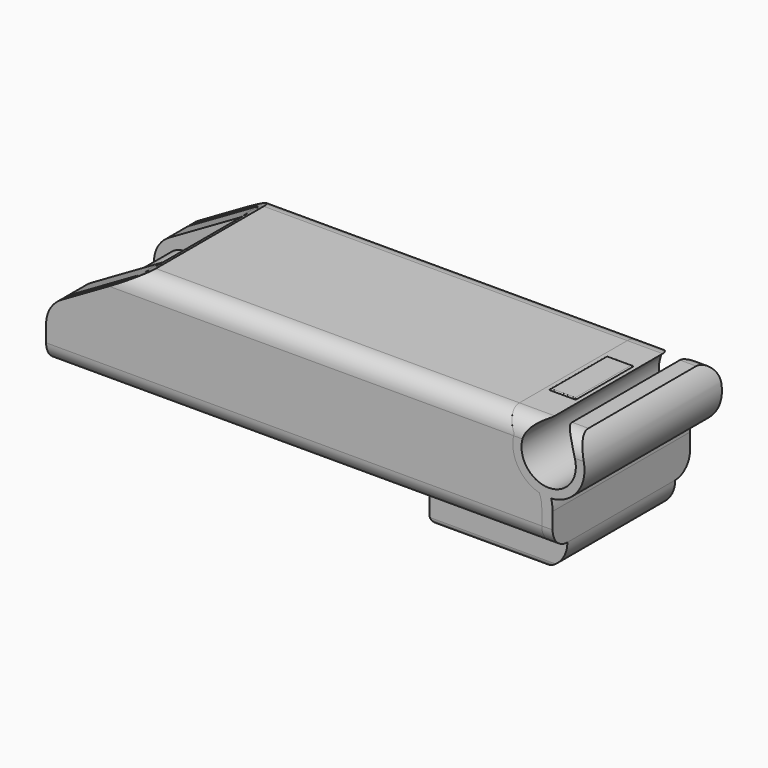
from build123d import *

# Parameters (mm, degrees)
F0_R      = 9
F1_DEPTH  = 65
F2_R      = 1.5
F2_2_R    = 1.5
F5_DEPTH  = 300
F0_R_2    = 16.5
F0_R_3    = 12.5
F6_DEPTH  = 12.5
F11_DEPTH = 400
F12_DEPTH = 300
F15_START = 25
F10_W     = 5
F10_H     = 1.1602536632
F15_DEPTH = 275
F16_DEPTH = 300
F17_R     = 12.5
F19_DEPTH = 79
F20_DEPTH = 300
F22_DEPTH = 0.5
F23_R     = 0.49999


# Not quite as in the source:
# - a fillet or chamfer is up to 0.001 mm smaller than in the source, because OpenCascade refuses the exact size
# - a feature names something its author has since deleted; it is built from what else it names


with BuildPart() as f1:
    # F0 (on Front) → F1 (new body)
    with BuildSketch(Plane.XZ):
        Circle(F0_R)
    extrude(amount=F1_DEPTH)

    # F2
    f2_edges = [f1.edges().sort_by_distance(p)[0] for p in [
        (-9, -65, 0),
        (-9, 0, 0),
    ]]
    fillet(f2_edges, radius=F2_R)


with BuildPart() as f1b:
    # F0 (on Front) → F1, piece 2 (new body)
    with BuildSketch(Plane.XZ):
        with Locations((30, 17.3205080757)):
            Circle(F0_R)
    extrude(amount=F1_DEPTH)

    # F2#2
    f2_2_edges = [f1b.edges().sort_by_distance(p)[0] for p in [
        (21, -65, 17.320508),
        (21, 0, 17.320508),
    ]]
    fillet(f2_2_edges, radius=F2_2_R)


with BuildPart() as f5:
    # F4 (on offset) → F5 (new body)
    with BuildSketch(Plane.YZ.offset(-50)):
        Polygon((-6.5, 31.1602540378), (-10, 31.1602540378), (-10, 8.6602540378), (-10, -13.8397459622), (-6.5, -13.8397459622), (-6.5, -12.8397459622), (-1.5, -12.8397459622), (-1.5, -13.8397459622), (2, -13.8397459622), (2, 8.6602540378), (2, 31.1602540378), (-1.5, 31.1602540378), (-1.5, 30.1602540378), (-6.5, 30.1602540378), align=None)
    extrude(amount=F5_DEPTH)

    # F0 (on Front) → F6 (cut, symmetric)
    with BuildSketch(Plane.XZ):
        with Locations((20, 0)):
            Circle(F0_R)
        with Locations((40, 0)):
            Circle(F0_R)
        Circle(F0_R)
        with Locations((60, 0)):
            Circle(F0_R)
        with Locations((30, 17.3205080757)):
            Circle(F0_R)
        with Locations((50, 17.3205080757)):
            Circle(F0_R)
        with Locations((80, 0)):
            Circle(F0_R)
        with Locations((70, 17.3205080757)):
            Circle(F0_R)
        with Locations((90, 17.3205080757)):
            Circle(F0_R)
        with Locations((100, 0)):
            Circle(F0_R)
        with Locations((120, 0)):
            Circle(F0_R)
        with Locations((110, 17.3205080757)):
            Circle(F0_R)
        with Locations((130, 17.3205080757)):
            Circle(F0_R)
        with Locations((140, 0)):
            Circle(F0_R)
        with Locations((160, 0)):
            Circle(F0_R)
        with Locations((150, 17.3205080757)):
            Circle(F0_R)
        with Locations((180, 0)):
            Circle(F0_R)
        with Locations((170, 17.3205080757)):
            Circle(F0_R)
        with Locations((190, 17.3205080757)):
            Circle(F0_R)
        with Locations((200, 0)):
            Circle(F0_R)
        with Locations((217.1852991866, 21.4689424953)):
            Circle(F0_R_2)
        with Locations((217.1852991866, 21.4689424953)):
            Circle(F0_R_3, mode=Mode.SUBTRACT)
        with Locations((217.1852991866, 21.4689424953)):
            Circle(F0_R_3)
    extrude(amount=F6_DEPTH, both=True, mode=Mode.SUBTRACT)


with BuildPart() as f9_1:
    # F9: instance of F5
    add(f5.part.mirror(Plane.XZ.offset(32.5)))


with BuildPart() as f11_tool:
    # F10 (on offset) → F11 (new body)
    with BuildSketch(Plane.YZ.offset(-50)):
        with BuildLine():
            Line((6.9999996253, -7.5), (6.9999996253, 24.8205080757))
            ThreePointArc((6.9999996253, 24.8205080757), (4.5104073752, 30.8309154508), (-1.5, 33.320507701))
            Line((-1.5, 33.320507701), (-63.5, 33.320507701))
            ThreePointArc((-63.5, 33.320507701), (-69.5104073752, 30.8309154508), (-71.9999996253, 24.8205080757))
            Line((-71.9999996253, 24.8205080757), (-71.9999996253, -7.5))
            ThreePointArc((-71.9999996253, -7.5), (-69.5104073752, -13.5104073752), (-63.5, -15.9999996253))
            Line((-63.5, -15.9999996253), (-1.5, -15.9999996253))
            ThreePointArc((-1.5, -15.9999996253), (4.5104073752, -13.5104073752), (6.9999996253, -7.5))
        make_face()
        with BuildLine():
            Line((-58.5, -13.9999996253), (-63.5, -13.9999996253))
            ThreePointArc((-63.5, -13.9999996253), (-68.0961938128, -12.0961938128), (-69.9999996253, -7.5))
            Line((-69.9999996253, -7.5), (-69.9999996253, 24.8205080757))
            ThreePointArc((-69.9999996253, 24.8205080757), (-68.0961938128, 29.4167018885), (-63.5, 31.320507701))
            Line((-63.5, 31.320507701), (-58.5, 31.320507701))
            Line((-58.5, 31.320507701), (-6.5, 31.320507701))
            Line((-6.5, 31.320507701), (-1.5, 31.320507701))
            ThreePointArc((-1.5, 31.320507701), (3.0961938128, 29.4167018885), (4.9999996253, 24.8205080757))
            Line((4.9999996253, 24.8205080757), (4.9999996253, -7.5))
            ThreePointArc((4.9999996253, -7.5), (3.0961938128, -12.0961938128), (-1.5, -13.9999996253))
            Line((-1.5, -13.9999996253), (-6.5, -13.9999996253))
            Line((-6.5, -13.9999996253), (-58.5, -13.9999996253))
        make_face(mode=Mode.SUBTRACT)
    extrude(amount=F11_DEPTH)


with BuildPart() as f5_1:
    add(f5.part)

    # F11: cut by f11_tool
    add(f11_tool.part, mode=Mode.SUBTRACT)


with BuildPart() as f9_1_1:
    add(f9_1.part)

    # F11: cut by f11_tool
    add(f11_tool.part, mode=Mode.SUBTRACT)


with BuildPart() as f12:
    # F10 (on offset) → F12 (new body)
    with BuildSketch(Plane.YZ.offset(-50)):
        with BuildLine():
            Line((6.9999996253, -7.5), (6.9999996253, 24.8205080757))
            ThreePointArc((6.9999996253, 24.8205080757), (4.5104073752, 30.8309154508), (-1.5, 33.320507701))
            Line((-1.5, 33.320507701), (-63.5, 33.320507701))
            ThreePointArc((-63.5, 33.320507701), (-69.5104073752, 30.8309154508), (-71.9999996253, 24.8205080757))
            Line((-71.9999996253, 24.8205080757), (-71.9999996253, -7.5))
            ThreePointArc((-71.9999996253, -7.5), (-69.5104073752, -13.5104073752), (-63.5, -15.9999996253))
            Line((-63.5, -15.9999996253), (-1.5, -15.9999996253))
            ThreePointArc((-1.5, -15.9999996253), (4.5104073752, -13.5104073752), (6.9999996253, -7.5))
        make_face()
        with BuildLine():
            Line((-58.5, -13.9999996253), (-63.5, -13.9999996253))
            ThreePointArc((-63.5, -13.9999996253), (-68.0961938128, -12.0961938128), (-69.9999996253, -7.5))
            Line((-69.9999996253, -7.5), (-69.9999996253, 24.8205080757))
            ThreePointArc((-69.9999996253, 24.8205080757), (-68.0961938128, 29.4167018885), (-63.5, 31.320507701))
            Line((-63.5, 31.320507701), (-58.5, 31.320507701))
            Line((-58.5, 31.320507701), (-6.5, 31.320507701))
            Line((-6.5, 31.320507701), (-1.5, 31.320507701))
            ThreePointArc((-1.5, 31.320507701), (3.0961938128, 29.4167018885), (4.9999996253, 24.8205080757))
            Line((4.9999996253, 24.8205080757), (4.9999996253, -7.5))
            ThreePointArc((4.9999996253, -7.5), (3.0961938128, -12.0961938128), (-1.5, -13.9999996253))
            Line((-1.5, -13.9999996253), (-6.5, -13.9999996253))
            Line((-6.5, -13.9999996253), (-58.5, -13.9999996253))
        make_face(mode=Mode.SUBTRACT)
    extrude(amount=F12_DEPTH)

    # F10 (on offset) → F15 (join)
    with BuildSketch(Plane.YZ.offset(-50).offset(F15_START)):
        Polygon((-1.5, 31.320507701), (-6.5, 31.320507701), (-6.5, 31.1602540378), (-6.5, 30.1602540378), (-1.5, 30.1602540378), align=None)
        with Locations((-4, -13.4198727937)):
            Rectangle(F10_W, F10_H)
        with Locations((-61, -13.4198727937)):
            Rectangle(F10_W, F10_H)
        with Locations((-61, 30.7403808694)):
            Rectangle(F10_W, F10_H)
    extrude(amount=F15_DEPTH)


with BuildPart() as f16_tool:
    # F14 (on offset) → F16 (new body)
    with BuildSketch(Plane.XZ.offset(-200)):
        with BuildLine():
            Line((-7, 12.124355653), (23.6506350946, 29.8205080757))
            Line((23.6506350946, 29.8205080757), (-55, 29.8205080757))
            Line((-55, 29.8205080757), (-55, -12.5))
            Line((-55, -12.5), (-14, -12.5))
            Line((-14, -12.5), (-14, 0))
            ThreePointArc((-14, 0), (-12.124355653, 7), (-7, 12.124355653))
        make_face()
        Polygon((23.6506350946, 29.8205080757), (51.8805326081, 46.1190470043), (52.5611825287, 49.578758275), (-63.44614923, 49.578758275), (-63.44614923, -25.4550632089), (-14, -25.4550632089), (-14, -12.5), (-55, -12.5), (-55, 29.8205080757), align=None)
        with BuildLine():
            Line((269.0510749817, 49.578758275), (238.6852991866, 49.578758275))
            Line((238.6852991866, 49.578758275), (196.257725358, 49.578758275))
            Line((196.257725358, 49.578758275), (195.3648013201, 36.0283996168))
            Line((195.3648013201, 36.0283996168), (201.2658884128, 25.8074169523))
            ThreePointArc((201.2658884128, 25.8074169523), (200.7852865606, 19.6552209442), (202.5986078678, 13.7567160743))
            ThreePointArc((202.5986078678, 13.7567160743), (206.8741196746, 8.5875769981), (212.8539586736, 5.5475892438))
            ThreePointArc((212.8539586736, 5.5475892438), (213.7104963701, 2.8323646101), (214, 0))
            Line((214, 0), (214, -36.3099910319))
            Line((214, -36.3099910319), (269.0510749817, -36.3099910319))
            Line((269.0510749817, -36.3099910319), (269.0510749817, 49.578758275))
        make_face()
    extrude(amount=F16_DEPTH)


with BuildPart() as f5_2:
    add(f5_1.part)

    # F16: cut by f16_tool
    add(f16_tool.part, mode=Mode.SUBTRACT)


with BuildPart() as f9_1_2:
    add(f9_1_1.part)

    # F16: cut by f16_tool
    add(f16_tool.part, mode=Mode.SUBTRACT)


with BuildPart() as f12_1:
    add(f12.part)

    # F16: cut by f16_tool
    add(f16_tool.part, mode=Mode.SUBTRACT)


with BuildPart() as f19:
    # F17 (on face) → F19 (new body)
    with BuildSketch(Plane.XZ.offset(71.9999996253)):
        with BuildLine():
            Line((214, -15.9999996253), (201.6768403856, -15.9999996253))
            Line((201.6768403856, -15.9999996253), (155.4608300924, -15.9999996253))
            Line((155.4608300924, -15.9999996253), (155.4608300924, -24.9999996253))
            ThreePointArc((155.4608300924, -24.9999996253), (156.6324029677, -27.8284267501), (159.4608300924, -28.9999996253))
            Line((159.4608300924, -28.9999996253), (205.4608300924, -28.9999996253))
            ThreePointArc((205.4608300924, -28.9999996253), (215.0023547323, -25.3661814941), (219, -15.9712808038))
            Line((219, -15.9712808038), (219, -7.5))
            Line((219, -7.5), (219, 0))
            ThreePointArc((219, 0), (218.83124222, 2.5267204935), (218.3279666892, 5.0085563826))
            ThreePointArc((218.3279666892, 5.0085563826), (215.568342787, 5.0483623593), (212.8539586736, 5.5475892438))
            ThreePointArc((212.8539586736, 5.5475892438), (213.7104963701, 2.8323646101), (214, 0))
            Line((214, 0), (214, -7.5))
            Line((214, -7.5), (214, -15.9999996253))
        make_face()
        with BuildLine():
            Line((196.9282034466, 33.320507701), (201.2658884128, 25.8074169523))
            ThreePointArc((201.2658884128, 25.8074169523), (202.9798930983, 29.8627758189), (205.7052990919, 33.320507701))
            Line((205.7052990919, 33.320507701), (196.9282034466, 33.320507701))
        make_face()
        with BuildLine():
            ThreePointArc((201.0292783844, 24.8205080757), (203.1213614916, 12.8401733763), (212.8539586736, 5.5475892438))
            ThreePointArc((212.8539586736, 5.5475892438), (215.568342787, 5.0483623593), (218.3279666892, 5.0085563826))
            ThreePointArc((218.3279666892, 5.0085563826), (232.2553608369, 28.1878145626), (205.7052990919, 33.320507701))
            ThreePointArc((205.7052990919, 33.320507701), (202.9798930983, 29.8627758189), (201.2658884128, 25.8074169523))
            ThreePointArc((201.2658884128, 25.8074169523), (201.1399937991, 25.3157821099), (201.0292783844, 24.8205080757))
        make_face()
        with Locations((217.1852991866, 21.4689424953)):
            Circle(F17_R, mode=Mode.SUBTRACT)
    extrude(amount=-F19_DEPTH)

    # F18 (on offset) → F20 (cut)
    with BuildSketch(Plane.YZ.offset(-50)):
        with BuildLine():
            Line((30.3000003567, 12.124355653), (30.3000003567, 24.8205080757))
            ThreePointArc((30.3000003567, 24.8205080757), (20.985995894, 47.3065039696), (-1.5, 56.6205084324))
            Line((-1.5, 56.6205084324), (-63.5, 56.6205084324))
            ThreePointArc((-63.5, 56.6205084324), (-85.985995894, 47.3065039696), (-95.3000003567, 24.8205080757))
            Line((-95.3000003567, 24.8205080757), (-95.3000003567, 12.124355653))
            Line((-95.3000003567, 12.124355653), (-95.3000003567, 0))
            Line((-95.3000003567, 0), (-95.3000003567, -7.5))
            ThreePointArc((-95.3000003567, -7.5), (-85.985995894, -29.985995894), (-63.5, -39.3000003567))
            Line((-63.5, -39.3000003567), (-1.5, -39.3000003567))
            ThreePointArc((-1.5, -39.3000003567), (20.985995894, -29.985995894), (30.3000003567, -7.5))
            Line((30.3000003567, -7.5), (30.3000003567, 0))
            Line((30.3000003567, 0), (30.3000003567, 12.124355653))
        make_face()
        with BuildLine():
            ThreePointArc((-1.5, 33.320507701), (4.5104073752, 30.8309154508), (6.9999996253, 24.8205080757))
            Line((6.9999996253, 24.8205080757), (6.9999996253, 12.124355653))
            Line((6.9999996253, 12.124355653), (6.9999996253, 0))
            Line((6.9999996253, 0), (6.9999996253, -7.5))
            ThreePointArc((6.9999996253, -7.5), (4.5104073752, -13.5104073752), (-1.5, -15.9999996253))
            Line((-1.5, -15.9999996253), (-1.5, -26.4999996253))
            ThreePointArc((-1.5, -26.4999996253), (-2.232233047, -28.2677665783), (-4, -28.9999996253))
            Line((-4, -28.9999996253), (-61, -28.9999996253))
            ThreePointArc((-61, -28.9999996253), (-62.767766953, -28.2677665783), (-63.5, -26.4999996253))
            Line((-63.5, -26.4999996253), (-63.5, -15.9999996253))
            ThreePointArc((-63.5, -15.9999996253), (-69.5104073752, -13.5104073752), (-71.9999996253, -7.5))
            Line((-71.9999996253, -7.5), (-71.9999996253, 0))
            Line((-71.9999996253, 0), (-71.9999996253, 12.124355653))
            Line((-71.9999996253, 12.124355653), (-71.9999996253, 24.8205080757))
            ThreePointArc((-71.9999996253, 24.8205080757), (-69.5104073752, 30.8309154508), (-63.5, 33.320507701))
            Line((-63.5, 33.320507701), (-1.5, 33.320507701))
        make_face(mode=Mode.SUBTRACT)
    extrude(amount=F20_DEPTH, mode=Mode.SUBTRACT)


with BuildPart() as f22:
    # F21 (on face) → F22 (new body)
    with BuildSketch(Plane.XY.offset(33.320507701)):
        Polygon((211.2115852847, -16), (199.2115852847, -16), (199.2115852847, -32.5), (199.2115852847, -49), (211.2115852847, -49), (211.2115852847, -32.5), align=None)
    extrude(amount=F22_DEPTH)

    # F23 (radius 0.5 in the source; OpenCascade refuses exactly that, so slightly less here)
    f23_edges = [f22.edges().sort_by_distance(p)[0] for p in [
        (205.211585, -16, 33.820508),
        (199.211585, -32.5, 33.820508),
        (205.211585, -49, 33.820508),
        (211.211585, -32.5, 33.820508),
    ]]
    fillet(f23_edges, radius=F23_R)


solid = Compound([f1.part, f1b.part, f5_2.part, f9_1_2.part, f12_1.part, f19.part, f22.part])
